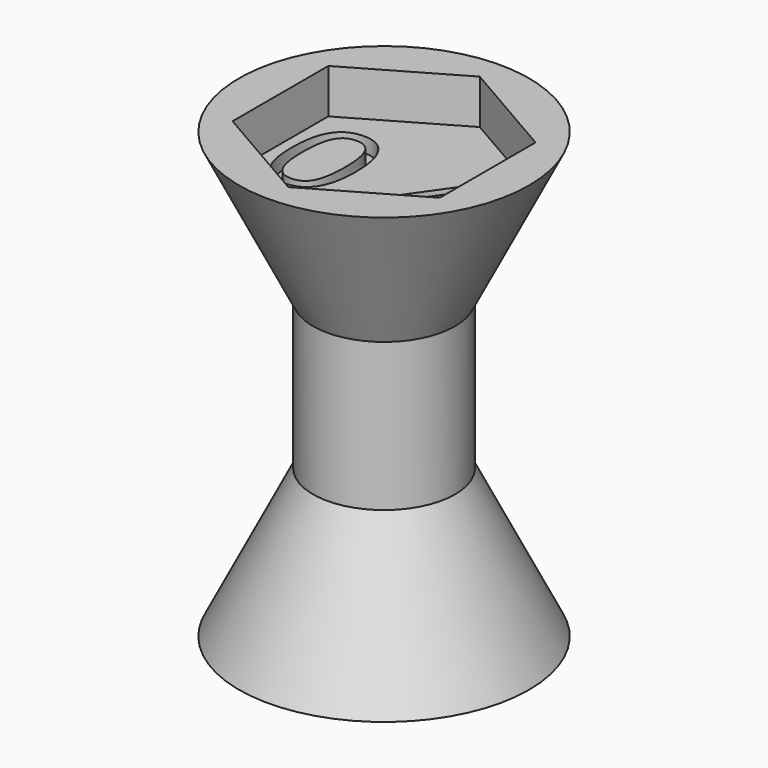
from build123d import *

# Parameters (mm, degrees)
F3_DEPTH     = 3
F4_TEXT_SIZE = 9.282337774
F5_DEPTH     = 1


# Not quite as in the source:
# - Text() gives the source's letters only with a copy of the font that has no kerning and outlines rounded to 1/6400 em; it was checked with that copy


with BuildPart() as f1:
    # F0 (on Front) → F1 (revolve)
    with BuildSketch(Plane.XZ):
        Polygon((9.8, 15), (0, 15), (0, -15), (9.8, -15), (4.8, -5), (4.8, 5), align=None)
    revolve(axis=Axis((0, 0, 0), (0, 0, -1)))

    # F2 (on face) → F3 (cut)
    with BuildSketch(Plane.XY.offset(15)):
        Polygon((7, 4.0414518843), (0, 8.0829037687), (-7, 4.0414518843), (-7, -4.0414518843), (0, -8.0829037687), (7, -4.0414518843), align=None)
    extrude(amount=-F3_DEPTH, mode=Mode.SUBTRACT)

    # F4 (on face) → F5 (cut)
    with BuildSketch(Plane.XY.offset(12)):
        with Locations((-6.75, -3.2750298711)):
            Text('0.4', F4_TEXT_SIZE, font='Open Sans', text_align=(TextAlign.LEFT, TextAlign.BOTTOM))
    extrude(amount=-F5_DEPTH, mode=Mode.SUBTRACT)


solid = f1.part
